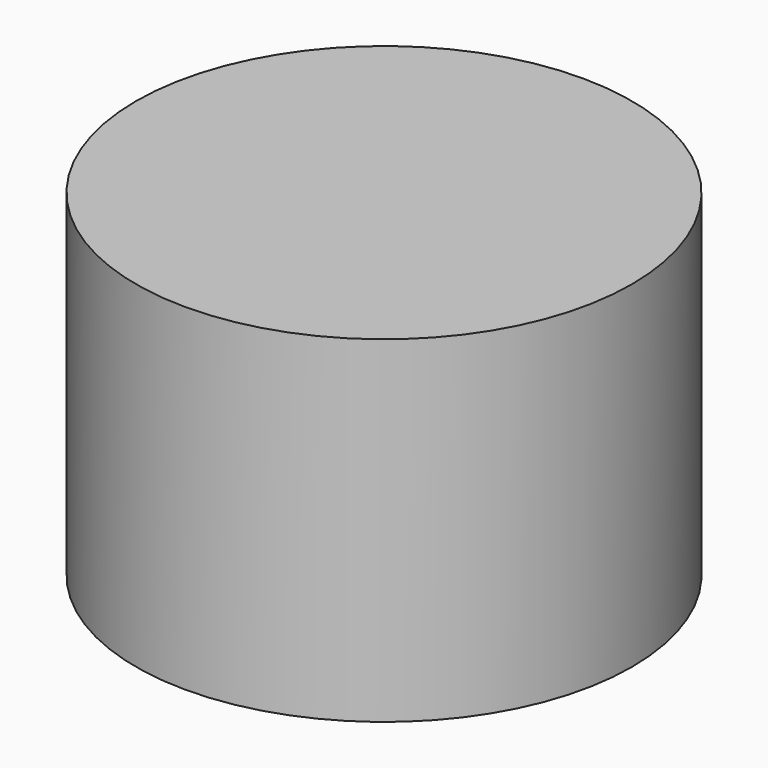
from build123d import *

# Parameters (mm, degrees)
F0_R     = 14.9546004533
F1_DEPTH = 20.32


# Not quite as in the source:
# - the program builds the solid bodies; features that only make, move or delete a surface that nothing else refers to are left out


with BuildPart() as f1:
    # F0 (on Top) → F1 (new body)
    with BuildSketch(Plane.XY):
        with Locations((6.7787659355, 5.6489733979)):
            Circle(F0_R)
    extrude(amount=-F1_DEPTH)


solid = f1.part
